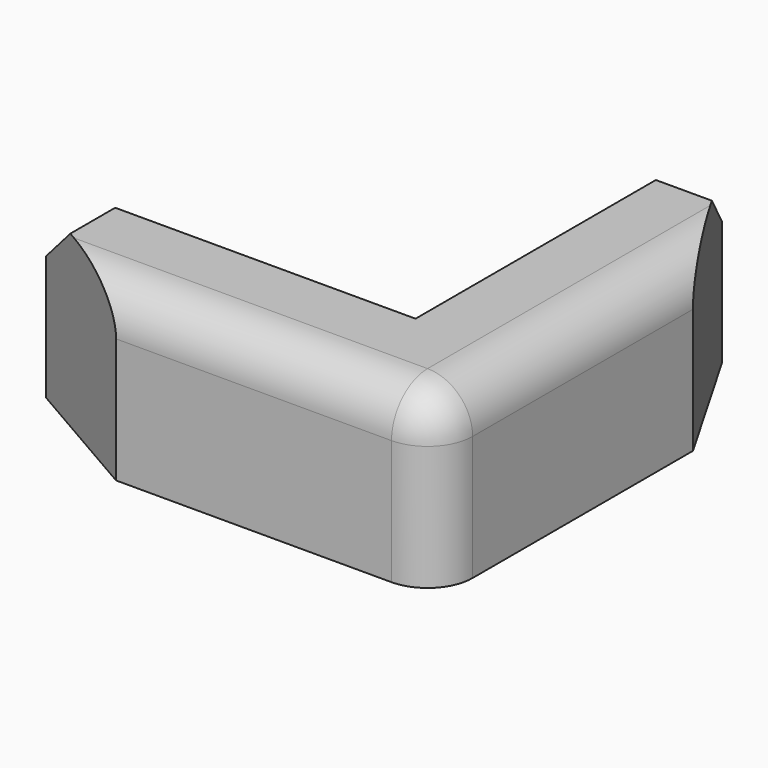
from build123d import *

# Parameters (mm, degrees)
F1_DEPTH     = 12.7
F0_W         = 50.8
F0_H         = 7.112
F2_DEPTH     = 25.4
F0_W_2       = 12.7
F0_H_2       = 21.59
F3_DEPTH     = 76.2
F4_DEPTH     = 76.2
F5_SIZE2     = 21.9970452561
F5_SIZE      = 12.7
F6_SIZE2     = 21.9970452561
F6_SIZE      = 12.7
F7_R         = 7.62
F8_T1_DEPTH  = 70.3962243683
F8_T3_DEPTH  = 70.3962243683
F8_T5_DEPTH  = 51.8924487366
F8_T7_DEPTH  = 51.8924487366
F8_T13_DEPTH = 89.9924487366
F8_T17_DEPTH = 89.9924487366


# Not quite as in the source:
# - a fillet or chamfer that OpenCascade refuses, or shapes differently, is made with other operations: its cross-section is extruded or revolved along the edge and cut away or added


with BuildPart() as f1:
    # F0 (on Front) → F1 (new body)
    with BuildSketch(Plane.XZ):
        Polygon((25.4, -14.351), (25.4, 7.239), (12.7, 7.239), (-38.1, 7.239), (-38.1, -14.351), align=None)
    extrude(amount=-F1_DEPTH)

    # F0 (on Front) → F2 (join)
    with BuildSketch(Plane.XZ):
        with Locations((-12.7, 10.795)):
            Rectangle(F0_W, F0_H)
    extrude(amount=-F2_DEPTH)

    # F0 (on Front) → F3 (join)
    with BuildSketch(Plane.XZ):
        with Locations((31.75, -3.556)):
            Rectangle(F0_W_2, F0_H_2)
        with Locations((31.75, 10.795)):
            Rectangle(F0_W_2, F0_H)
    extrude(amount=-F3_DEPTH)

    # F0 (on Front) → F4 (join)
    with BuildSketch(Plane.XZ):
        with Locations((19.05, 10.795)):
            Rectangle(F0_W_2, F0_H)
    extrude(amount=-F4_DEPTH)

    # F5
    f5_edges = [f1.edges().sort_by_distance(p)[0] for p in [
        (38.1, 76.2, 0),
    ]]
    f5_side = f1.faces().sort_by_distance((29.228014, 76.2, 2.143688))[0]
    chamfer(f5_edges, length=F5_SIZE, length2=F5_SIZE2, reference=f5_side)

    # F6
    f6_edges = [f1.edges().sort_by_distance(p)[0] for p in [
        (-38.1, 0, 0),
    ]]
    chamfer(f6_edges, length=F6_SIZE, length2=F6_SIZE2)

    # F7
    f7_edges = [f1.edges().sort_by_distance(p)[0] for p in [
        (38.1, 27.101477, 14.351),
        (10.998523, 0, 14.351),
        (38.1, 0, 0),
    ]]
    fillet(f7_edges, radius=F7_R)

    # F8: chamfer of 7.62 on 4 edges, made by hand

    # F8_s2 → F8_t1 (cut)
    with BuildSketch(Plane.YZ.offset(-57.6962243683)):
        Polygon((17.78, 14.351), (25.4, 6.731), (25.4, 14.351), align=None)
    extrude(amount=F8_T1_DEPTH, mode=Mode.SUBTRACT)

    # F8_s4 → F8_t3 (cut)
    with BuildSketch(Plane.XZ.offset(-95.7962243683)):
        Polygon((20.32, 14.351), (12.7, 6.731), (12.7, 14.351), align=None)
    extrude(amount=F8_T3_DEPTH, mode=Mode.SUBTRACT)

    # F8_s6 → F8_t5 (cut)
    with BuildSketch(Plane.YZ.offset(-6.8962243683)):
        Polygon((68.58, 14.351), (76.2, 6.731), (76.2, 14.351), align=None)
    extrude(amount=F8_T5_DEPTH, mode=Mode.SUBTRACT)

    # F8_s8 → F8_t7 (cut)
    with BuildSketch(Plane.XZ.offset(-44.9962243683)):
        Polygon((-30.48, 14.351), (-38.1, 6.731), (-38.1, 14.351), align=None)
    extrude(amount=F8_T7_DEPTH, mode=Mode.SUBTRACT)


with BuildPart() as f8_tool11:
    # F8_s12 → F8_t13 (new body)
    with BuildSketch(Plane.YZ.offset(32.2962243683)):
        Polygon((17.78, 14.351), (25.4, 6.731), (25.4, 14.351), align=None)
    extrude(amount=-F8_T13_DEPTH)

    split(bisect_by=Plane.YZ.offset(12.7), keep=Keep.TOP)


with BuildPart() as f8_tool15:
    # F8_s16 → F8_t17 (new body)
    with BuildSketch(Plane.XZ.offset(-5.8037756317)):
        Polygon((20.32, 14.351), (12.7, 6.731), (12.7, 14.351), align=None)
    extrude(amount=-F8_T17_DEPTH)

    split(bisect_by=Plane.XZ.offset(-25.4), keep=Keep.TOP)


with BuildPart() as f8_tool11_1:
    add(f8_tool11.part)

    # F8_t19: intersect F8_tool15
    add(f8_tool15.part, mode=Mode.INTERSECT)


with BuildPart() as f1_1:
    add(f1.part)

    # F8_t9: cut F8_tool11
    add(f8_tool11_1.part, mode=Mode.SUBTRACT)


solid = f1_1.part
